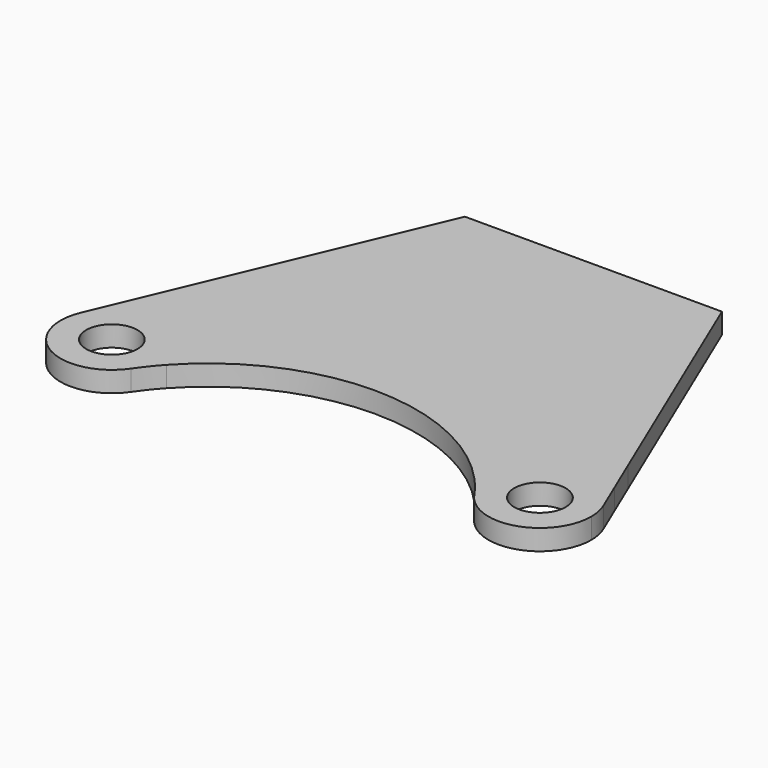
from build123d import *

# Parameters (mm, degrees)
F0_R     = 10
F1_DEPTH = 8


with BuildPart() as f1:
    # F0 (on Top) → F1 (new body)
    with BuildSketch(Plane.XY):
        with BuildLine():
            ThreePointArc((66.8107155763, 68.8983527146), (89.2220086446, 61.1485010982), (103.2801650714, 80.2454771665))
            ThreePointArc((103.2801650714, 80.2454771665), (102.8817929615, 84.2174016446), (101.7025466654, 88.0310957293))
            ThreePointArc((101.7025466654, 88.0310957293), (73.6640874011, 97.7820404055), (66.8107155763, 68.8983527146))
        make_face()
        with Locations((83.2801650714, 80.2454771665)):
            Circle(F0_R, mode=Mode.SUBTRACT)
        with BuildLine():
            ThreePointArc((66.8107155763, 68.8983527146), (73.6640874011, 97.7820404055), (101.7025466654, 88.0310957293))
            Line((101.7025466654, 88.0310957293), (96.8992238213, 99.3967496769))
            ThreePointArc((96.8992238213, 99.3967496769), (71.3236564608, 100.476441104), (59.9351524158, 77.550967172))
            ThreePointArc((59.9351524158, 77.550967172), (63.5204352748, 73.3418677958), (66.8107155763, 68.8983527146))
        make_face()
        with BuildLine():
            ThreePointArc((59.9351524158, 77.550967172), (71.3236564608, 100.476441104), (96.8992238213, 99.3967496769))
            Line((96.8992238213, 99.3967496769), (90.8352022654, 113.7454771665))
            Line((90.8352022654, 113.7454771665), (-90.8352022654, 113.7454771665))
            Line((-90.8352022654, 113.7454771665), (-96.8992238213, 99.3967496769))
            ThreePointArc((-96.8992238213, 99.3967496769), (-72.5051449003, 101.1296563534), (-59.7801650714, 80.2454771665))
            ThreePointArc((-59.7801650714, 80.2454771665), (-59.8189439032, 78.8959953041), (-59.9351524158, 77.550967172))
            ThreePointArc((-59.9351524158, 77.550967172), (0, 104), (59.9351524158, 77.550967172))
        make_face()
        with BuildLine():
            ThreePointArc((-66.8107155763, 68.8983527146), (-63.5204352748, 73.3418677958), (-59.9351524158, 77.550967172))
            ThreePointArc((-59.9351524158, 77.550967172), (-59.8189439032, 78.8959953041), (-59.7801650714, 80.2454771665))
            ThreePointArc((-59.7801650714, 80.2454771665), (-72.5051449003, 101.1296563534), (-96.8992238213, 99.3967496769))
            Line((-96.8992238213, 99.3967496769), (-101.7025466654, 88.0310957293))
            ThreePointArc((-101.7025466654, 88.0310957293), (-79.3082405933, 99.8471050565), (-63.2801650714, 80.2454771665))
            ThreePointArc((-63.2801650714, 80.2454771665), (-64.1831890032, 74.3036335933), (-66.8107155763, 68.8983527146))
        make_face()
        with BuildLine():
            ThreePointArc((-101.7025466654, 88.0310957293), (-92.8962427418, 62.7089139274), (-66.8107155763, 68.8983527146))
            ThreePointArc((-66.8107155763, 68.8983527146), (-64.1831890032, 74.3036335933), (-63.2801650714, 80.2454771665))
            ThreePointArc((-63.2801650714, 80.2454771665), (-79.3082405933, 99.8471050565), (-101.7025466654, 88.0310957293))
        make_face()
        with Locations((-83.2801650714, 80.2454771665)):
            Circle(F0_R, mode=Mode.SUBTRACT)
        Polygon((-90.8352022654, 113.7454771665), (90.8352022654, 113.7454771665), (50, 210.37), (0, 210.37), (-50, 210.37), align=None)
    extrude(amount=F1_DEPTH)


solid = f1.part
